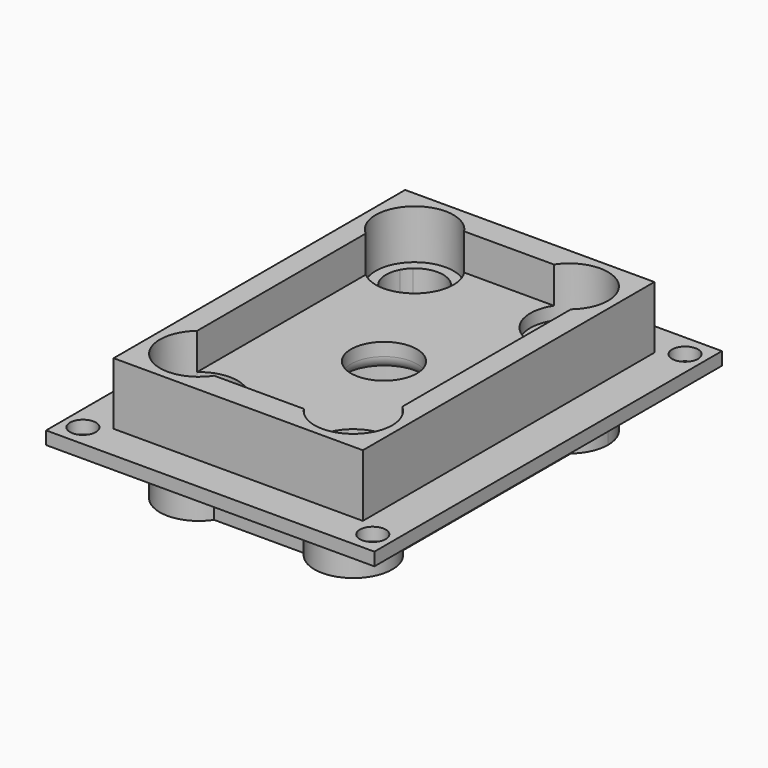
from build123d import *

# Parameters (mm, degrees)
F0_W      = 96.2
F0_H      = 140.65
F0_R      = 12.7
F1_DEPTH  = 5
F2_DEPTH  = 5
F3_DEPTH  = 19
F4_W      = 126.71781471
F4_H      = 167.6731868647
F4_R      = 5
F4_W_2    = 96.2
F4_H_2    = 140.65
F4_R_2    = 11
F4_R_3    = 30
F2_FACE_R = 12.7
F5_DEPTH  = 5
F6_DEPTH  = 30
F7_DEPTH  = 25
F8_R      = 12.7
F9_DEPTH  = 35
F4_R_4    = 12.7
F10_DEPTH = 35
F11_R     = 4.99999


# Not quite as in the source:
# - a fillet or chamfer is up to 0.001 mm smaller than in the source, because OpenCascade refuses the exact size


with BuildPart() as f1:
    # F0 (on Top) → F1 (new body)
    with BuildSketch(Plane.XY):
        with Locations((-2.6661262382, -2.1749504376)):
            Rectangle(F0_W, F0_H)
        with BuildLine():
            ThreePointArc((-42.2661262382, 38.498499743), (-42.4198102031, 61.1325113488), (-19.9826307497, 58.1500495624))
            Line((-19.9826307497, 58.1500495624), (14.6503782733, 58.1500495624))
            ThreePointArc((14.6503782733, 58.1500495624), (31.4825998108, 64.2478800491), (42.1661737618, 49.8823495624))
            ThreePointArc((42.1661737618, 49.8823495624), (40.7954712492, 43.6179860672), (36.9338737618, 38.498499743))
            Line((36.9338737618, 38.498499743), (36.9338737618, -42.8484006182))
            ThreePointArc((36.9338737618, -42.8484006182), (40.7954712492, -47.9678869424), (42.1661737618, -54.2322504376))
            ThreePointArc((42.1661737618, -54.2322504376), (31.4825998108, -68.5977809243), (14.6503782733, -62.4999504376))
            Line((14.6503782733, -62.4999504376), (-19.9826307497, -62.4999504376))
            ThreePointArc((-19.9826307497, -62.4999504376), (-42.4198102031, -65.482412224), (-42.2661262382, -42.8484006182))
            Line((-42.2661262382, -42.8484006182), (-42.2661262382, 38.498499743))
        make_face(mode=Mode.SUBTRACT)
        with BuildLine():
            Line((14.6503782733, 58.1500495624), (-19.9826307497, 58.1500495624))
            ThreePointArc((-19.9826307497, 58.1500495624), (-18.1328957515, 54.1987756114), (-17.4984262382, 49.8823495624))
            ThreePointArc((-17.4984262382, 49.8823495624), (-26.234062743, 36.253052075), (-42.2661262382, 38.498499743))
            Line((-42.2661262382, 38.498499743), (-42.2661262382, -42.8484006182))
            ThreePointArc((-42.2661262382, -42.8484006182), (-26.234062743, -40.6029529502), (-17.4984262382, -54.2322504376))
            ThreePointArc((-17.4984262382, -54.2322504376), (-18.1328957515, -58.5486764866), (-19.9826307497, -62.4999504376))
            Line((-19.9826307497, -62.4999504376), (14.6503782733, -62.4999504376))
            ThreePointArc((14.6503782733, -62.4999504376), (17.2447897969, -42.9820886512), (36.9338737618, -42.8484006182))
            Line((36.9338737618, -42.8484006182), (36.9338737618, 38.498499743))
            ThreePointArc((36.9338737618, 38.498499743), (17.2447897969, 38.632187776), (14.6503782733, 58.1500495624))
        make_face()
        with Locations((-2.6661262382, -2.1749504376)):
            Circle(F0_R, mode=Mode.SUBTRACT)
        with BuildLine():
            Line((-19.9826307497, 58.1500495624), (-25.2427293929, 58.1500495624))
            ThreePointArc((-25.2427293929, 58.1500495624), (-22.4781302022, 54.4203741713), (-21.4984262382, 49.8823495624))
            ThreePointArc((-21.4984262382, 49.8823495624), (-29.8950342201, 39.1948638899), (-42.2661262382, 44.823492309))
            Line((-42.2661262382, 44.823492309), (-42.2661262382, 38.498499743))
            ThreePointArc((-42.2661262382, 38.498499743), (-26.234062743, 36.253052075), (-17.4984262382, 49.8823495624))
            ThreePointArc((-17.4984262382, 49.8823495624), (-18.1328957515, 54.1987756114), (-19.9826307497, 58.1500495624))
        make_face()
        with BuildLine():
            Line((19.9104769166, 58.1500495624), (14.6503782733, 58.1500495624))
            ThreePointArc((14.6503782733, 58.1500495624), (17.2447897969, 38.632187776), (36.9338737618, 38.498499743))
            Line((36.9338737618, 38.498499743), (36.9338737618, 44.823492309))
            ThreePointArc((36.9338737618, 44.823492309), (20.3855526974, 41.2207574466), (19.9104769166, 58.1500495624))
        make_face()
        with BuildLine():
            ThreePointArc((-17.4984262382, -54.2322504376), (-26.234062743, -40.6029529502), (-42.2661262382, -42.8484006182))
            Line((-42.2661262382, -42.8484006182), (-42.2661262382, -49.1733931842))
            ThreePointArc((-42.2661262382, -49.1733931842), (-29.8950342201, -43.5447647651), (-21.4984262382, -54.2322504376))
            ThreePointArc((-21.4984262382, -54.2322504376), (-22.4781302022, -58.7702750465), (-25.2427293929, -62.4999504376))
            Line((-25.2427293929, -62.4999504376), (-19.9826307497, -62.4999504376))
            ThreePointArc((-19.9826307497, -62.4999504376), (-18.1328957515, -58.5486764866), (-17.4984262382, -54.2322504376))
        make_face()
        with BuildLine():
            Line((36.9338737618, -49.1733931842), (36.9338737618, -42.8484006182))
            ThreePointArc((36.9338737618, -42.8484006182), (17.2447897969, -42.9820886512), (14.6503782733, -62.4999504376))
            Line((14.6503782733, -62.4999504376), (19.9104769166, -62.4999504376))
            ThreePointArc((19.9104769166, -62.4999504376), (20.3855526974, -45.5706583218), (36.9338737618, -49.1733931842))
        make_face()
        with BuildLine():
            Line((-42.2661262382, 54.9412068158), (-42.2661262382, 58.1500495624))
            Line((-42.2661262382, 58.1500495624), (-39.7541230834, 58.1500495624))
            ThreePointArc((-39.7541230834, 58.1500495624), (-32.4984262382, 60.8823495624), (-25.2427293929, 58.1500495624))
            Line((-25.2427293929, 58.1500495624), (-19.9826307497, 58.1500495624))
            ThreePointArc((-19.9826307497, 58.1500495624), (-42.4198102031, 61.1325113488), (-42.2661262382, 38.498499743))
            Line((-42.2661262382, 38.498499743), (-42.2661262382, 44.823492309))
            ThreePointArc((-42.2661262382, 44.823492309), (-43.4984262382, 49.8823495624), (-42.2661262382, 54.9412068158))
        make_face()
        with BuildLine():
            ThreePointArc((42.1661737618, 49.8823495624), (31.4825998108, 64.2478800491), (14.6503782733, 58.1500495624))
            Line((14.6503782733, 58.1500495624), (19.9104769166, 58.1500495624))
            ThreePointArc((19.9104769166, 58.1500495624), (27.1661737618, 60.8823495624), (34.4218706071, 58.1500495624))
            Line((34.4218706071, 58.1500495624), (36.9338737618, 58.1500495624))
            Line((36.9338737618, 58.1500495624), (36.9338737618, 54.9412068158))
            ThreePointArc((36.9338737618, 54.9412068158), (37.8536594343, 52.4857415805), (38.1661737618, 49.8823495624))
            ThreePointArc((38.1661737618, 49.8823495624), (37.8536594343, 47.2789575443), (36.9338737618, 44.823492309))
            Line((36.9338737618, 44.823492309), (36.9338737618, 38.498499743))
            ThreePointArc((36.9338737618, 38.498499743), (40.7954712492, 43.6179860672), (42.1661737618, 49.8823495624))
        make_face()
        with BuildLine():
            Line((-42.2661262382, -49.1733931842), (-42.2661262382, -42.8484006182))
            ThreePointArc((-42.2661262382, -42.8484006182), (-42.4198102031, -65.482412224), (-19.9826307497, -62.4999504376))
            Line((-19.9826307497, -62.4999504376), (-25.2427293929, -62.4999504376))
            ThreePointArc((-25.2427293929, -62.4999504376), (-32.4984262382, -65.2322504376), (-39.7541230834, -62.4999504376))
            Line((-39.7541230834, -62.4999504376), (-42.2661262382, -62.4999504376))
            Line((-42.2661262382, -62.4999504376), (-42.2661262382, -59.291107691))
            ThreePointArc((-42.2661262382, -59.291107691), (-43.4984262382, -54.2322504376), (-42.2661262382, -49.1733931842))
        make_face()
        with BuildLine():
            ThreePointArc((42.1661737618, -54.2322504376), (40.7954712492, -47.9678869424), (36.9338737618, -42.8484006182))
            Line((36.9338737618, -42.8484006182), (36.9338737618, -49.1733931842))
            ThreePointArc((36.9338737618, -49.1733931842), (37.8536594343, -51.6288584195), (38.1661737618, -54.2322504376))
            ThreePointArc((38.1661737618, -54.2322504376), (37.8536594343, -56.8356424557), (36.9338737618, -59.291107691))
            Line((36.9338737618, -59.291107691), (36.9338737618, -62.4999504376))
            Line((36.9338737618, -62.4999504376), (34.4218706071, -62.4999504376))
            ThreePointArc((34.4218706071, -62.4999504376), (27.1661737618, -65.2322504376), (19.9104769166, -62.4999504376))
            Line((19.9104769166, -62.4999504376), (14.6503782733, -62.4999504376))
            ThreePointArc((14.6503782733, -62.4999504376), (31.4825998108, -68.5977809243), (42.1661737618, -54.2322504376))
        make_face()
        with BuildLine():
            Line((36.9338737618, 58.1500495624), (34.4218706071, 58.1500495624))
            ThreePointArc((34.4218706071, 58.1500495624), (35.8277658776, 56.6629706268), (36.9338737618, 54.9412068158))
            Line((36.9338737618, 54.9412068158), (36.9338737618, 58.1500495624))
        make_face()
        with BuildLine():
            Line((-39.7541230834, 58.1500495624), (-42.2661262382, 58.1500495624))
            Line((-42.2661262382, 58.1500495624), (-42.2661262382, 54.9412068158))
            ThreePointArc((-42.2661262382, 54.9412068158), (-41.160018354, 56.6629706268), (-39.7541230834, 58.1500495624))
        make_face()
        with BuildLine():
            Line((36.9338737618, -62.4999504376), (36.9338737618, -59.291107691))
            ThreePointArc((36.9338737618, -59.291107691), (35.8277658776, -61.012871502), (34.4218706071, -62.4999504376))
            Line((34.4218706071, -62.4999504376), (36.9338737618, -62.4999504376))
        make_face()
        with BuildLine():
            ThreePointArc((-39.7541230834, -62.4999504376), (-41.160018354, -61.012871502), (-42.2661262382, -59.291107691))
            Line((-42.2661262382, -59.291107691), (-42.2661262382, -62.4999504376))
            Line((-42.2661262382, -62.4999504376), (-39.7541230834, -62.4999504376))
        make_face()
    extrude(amount=-F1_DEPTH)

    # F0 (on Top) → F2 (join)
    with BuildSketch(Plane.XY):
        with BuildLine():
            Line((14.6503782733, 58.1500495624), (-19.9826307497, 58.1500495624))
            ThreePointArc((-19.9826307497, 58.1500495624), (-18.1328957515, 54.1987756114), (-17.4984262382, 49.8823495624))
            ThreePointArc((-17.4984262382, 49.8823495624), (-26.234062743, 36.253052075), (-42.2661262382, 38.498499743))
            Line((-42.2661262382, 38.498499743), (-42.2661262382, -42.8484006182))
            ThreePointArc((-42.2661262382, -42.8484006182), (-26.234062743, -40.6029529502), (-17.4984262382, -54.2322504376))
            ThreePointArc((-17.4984262382, -54.2322504376), (-18.1328957515, -58.5486764866), (-19.9826307497, -62.4999504376))
            Line((-19.9826307497, -62.4999504376), (14.6503782733, -62.4999504376))
            ThreePointArc((14.6503782733, -62.4999504376), (17.2447897969, -42.9820886512), (36.9338737618, -42.8484006182))
            Line((36.9338737618, -42.8484006182), (36.9338737618, 38.498499743))
            ThreePointArc((36.9338737618, 38.498499743), (17.2447897969, 38.632187776), (14.6503782733, 58.1500495624))
        make_face()
        with Locations((-2.6661262382, -2.1749504376)):
            Circle(F0_R, mode=Mode.SUBTRACT)
    extrude(amount=F2_DEPTH)

    # F0 (on Top) → F3 (join)
    with BuildSketch(Plane.XY):
        with Locations((-2.6661262382, -2.1749504376)):
            Rectangle(F0_W, F0_H)
        with BuildLine():
            ThreePointArc((-42.2661262382, 38.498499743), (-42.4198102031, 61.1325113488), (-19.9826307497, 58.1500495624))
            Line((-19.9826307497, 58.1500495624), (14.6503782733, 58.1500495624))
            ThreePointArc((14.6503782733, 58.1500495624), (31.4825998108, 64.2478800491), (42.1661737618, 49.8823495624))
            ThreePointArc((42.1661737618, 49.8823495624), (40.7954712492, 43.6179860672), (36.9338737618, 38.498499743))
            Line((36.9338737618, 38.498499743), (36.9338737618, -42.8484006182))
            ThreePointArc((36.9338737618, -42.8484006182), (40.7954712492, -47.9678869424), (42.1661737618, -54.2322504376))
            ThreePointArc((42.1661737618, -54.2322504376), (31.4825998108, -68.5977809243), (14.6503782733, -62.4999504376))
            Line((14.6503782733, -62.4999504376), (-19.9826307497, -62.4999504376))
            ThreePointArc((-19.9826307497, -62.4999504376), (-42.4198102031, -65.482412224), (-42.2661262382, -42.8484006182))
            Line((-42.2661262382, -42.8484006182), (-42.2661262382, 38.498499743))
        make_face(mode=Mode.SUBTRACT)
    extrude(amount=F3_DEPTH)

    # F4 (on face) + F2_face (on face) → F5 (join)
    with BuildSketch(Plane(origin=(0, 0, -5), x_dir=(1, 0, 0), z_dir=(0, 0, -1))):
        with Locations((-2.6661262382, 2.1749504376)):
            Rectangle(F4_W, F4_H)
        with Locations((-58.5996061093, -73.1500495624)):
            Circle(F4_R, mode=Mode.SUBTRACT)
        with Locations((53.2673536329, -73.1500495624)):
            Circle(F4_R, mode=Mode.SUBTRACT)
        with Locations((-2.6661262382, 2.1749504376)):
            Rectangle(F4_W_2, F4_H_2, mode=Mode.SUBTRACT)
        with Locations((-58.5996061093, 77.4999504376)):
            Circle(F4_R, mode=Mode.SUBTRACT)
        with Locations((53.2673536329, 77.4999504376)):
            Circle(F4_R, mode=Mode.SUBTRACT)
        with Locations((-2.6661262382, 2.1749504376)):
            Rectangle(F4_W_2, F4_H_2)
        with Locations((-32.4984262382, -49.8823495624)):
            Circle(F4_R_2, mode=Mode.SUBTRACT)
        with Locations((27.1661737618, -49.8823495624)):
            Circle(F4_R_2, mode=Mode.SUBTRACT)
        with Locations((-32.4984262382, 54.2322504376)):
            Circle(F4_R_2, mode=Mode.SUBTRACT)
        with Locations((-2.6661262382, 2.1749504376)):
            Circle(F4_R_3, mode=Mode.SUBTRACT)
        with Locations((27.1661737618, 54.2322504376)):
            Circle(F4_R_2, mode=Mode.SUBTRACT)
    with BuildSketch(Plane(origin=(-2.6661262382, -2.1749504376, 5), x_dir=(1, 0, 0), z_dir=(0, 0, 1))):
        with BuildLine():
            Line((17.3165045115, 60.325), (-17.3165045115, 60.325))
            ThreePointArc((-17.3165045115, 60.325), (-19.9109160351, 40.8071382136), (-39.6, 40.6734501806))
            Line((-39.6, 40.6734501806), (-39.6, -40.6734501806))
            ThreePointArc((-39.6, -40.6734501806), (-19.9109160351, -40.8071382136), (-17.3165045115, -60.325))
            Line((-17.3165045115, -60.325), (17.3165045115, -60.325))
            ThreePointArc((17.3165045115, -60.325), (19.9109160351, -40.8071382136), (39.6, -40.6734501806))
            Line((39.6, -40.6734501806), (39.6, 40.6734501806))
            ThreePointArc((39.6, 40.6734501806), (19.9109160351, 40.8071382136), (17.3165045115, 60.325))
        make_face()
        Circle(F2_FACE_R, mode=Mode.SUBTRACT)
    extrude(amount=F5_DEPTH, dir=(0, 0, -1))

    # F0 (on Top) → F6 (join)
    with BuildSketch(Plane.XY):
        with BuildLine():
            Line((-42.2661262382, 54.9412068158), (-42.2661262382, 58.1500495624))
            Line((-42.2661262382, 58.1500495624), (-39.7541230834, 58.1500495624))
            ThreePointArc((-39.7541230834, 58.1500495624), (-32.4984262382, 60.8823495624), (-25.2427293929, 58.1500495624))
            Line((-25.2427293929, 58.1500495624), (-19.9826307497, 58.1500495624))
            ThreePointArc((-19.9826307497, 58.1500495624), (-42.4198102031, 61.1325113488), (-42.2661262382, 38.498499743))
            Line((-42.2661262382, 38.498499743), (-42.2661262382, 44.823492309))
            ThreePointArc((-42.2661262382, 44.823492309), (-43.4984262382, 49.8823495624), (-42.2661262382, 54.9412068158))
        make_face()
        with BuildLine():
            ThreePointArc((-25.2427293929, 58.1500495624), (-32.4984262382, 60.8823495624), (-39.7541230834, 58.1500495624))
            Line((-39.7541230834, 58.1500495624), (-25.2427293929, 58.1500495624))
        make_face()
        with BuildLine():
            Line((-39.7541230834, 58.1500495624), (-42.2661262382, 58.1500495624))
            Line((-42.2661262382, 58.1500495624), (-42.2661262382, 54.9412068158))
            ThreePointArc((-42.2661262382, 54.9412068158), (-41.160018354, 56.6629706268), (-39.7541230834, 58.1500495624))
        make_face()
        with BuildLine():
            Line((-42.2661262382, 44.823492309), (-42.2661262382, 54.9412068158))
            ThreePointArc((-42.2661262382, 54.9412068158), (-43.4984262382, 49.8823495624), (-42.2661262382, 44.823492309))
        make_face()
        with BuildLine():
            Line((-19.9826307497, 58.1500495624), (-25.2427293929, 58.1500495624))
            ThreePointArc((-25.2427293929, 58.1500495624), (-22.4781302022, 54.4203741713), (-21.4984262382, 49.8823495624))
            ThreePointArc((-21.4984262382, 49.8823495624), (-29.8950342201, 39.1948638899), (-42.2661262382, 44.823492309))
            Line((-42.2661262382, 44.823492309), (-42.2661262382, 38.498499743))
            ThreePointArc((-42.2661262382, 38.498499743), (-26.234062743, 36.253052075), (-17.4984262382, 49.8823495624))
            ThreePointArc((-17.4984262382, 49.8823495624), (-18.1328957515, 54.1987756114), (-19.9826307497, 58.1500495624))
        make_face()
        with BuildLine():
            Line((-25.2427293929, 58.1500495624), (-39.7541230834, 58.1500495624))
            ThreePointArc((-39.7541230834, 58.1500495624), (-41.160018354, 56.6629706268), (-42.2661262382, 54.9412068158))
            Line((-42.2661262382, 54.9412068158), (-42.2661262382, 44.823492309))
            ThreePointArc((-42.2661262382, 44.823492309), (-29.8950342201, 39.1948638899), (-21.4984262382, 49.8823495624))
            ThreePointArc((-21.4984262382, 49.8823495624), (-22.4781302022, 54.4203741713), (-25.2427293929, 58.1500495624))
        make_face()
        with BuildLine():
            ThreePointArc((42.1661737618, 49.8823495624), (31.4825998108, 64.2478800491), (14.6503782733, 58.1500495624))
            Line((14.6503782733, 58.1500495624), (19.9104769166, 58.1500495624))
            ThreePointArc((19.9104769166, 58.1500495624), (27.1661737618, 60.8823495624), (34.4218706071, 58.1500495624))
            Line((34.4218706071, 58.1500495624), (36.9338737618, 58.1500495624))
            Line((36.9338737618, 58.1500495624), (36.9338737618, 54.9412068158))
            ThreePointArc((36.9338737618, 54.9412068158), (37.8536594343, 52.4857415805), (38.1661737618, 49.8823495624))
            ThreePointArc((38.1661737618, 49.8823495624), (37.8536594343, 47.2789575443), (36.9338737618, 44.823492309))
            Line((36.9338737618, 44.823492309), (36.9338737618, 38.498499743))
            ThreePointArc((36.9338737618, 38.498499743), (40.7954712492, 43.6179860672), (42.1661737618, 49.8823495624))
        make_face()
        with BuildLine():
            Line((36.9338737618, 54.9412068158), (36.9338737618, 44.823492309))
            ThreePointArc((36.9338737618, 44.823492309), (37.8536594343, 47.2789575443), (38.1661737618, 49.8823495624))
            ThreePointArc((38.1661737618, 49.8823495624), (37.8536594343, 52.4857415805), (36.9338737618, 54.9412068158))
        make_face()
        with BuildLine():
            Line((34.4218706071, 58.1500495624), (19.9104769166, 58.1500495624))
            ThreePointArc((19.9104769166, 58.1500495624), (20.3855526974, 41.2207574466), (36.9338737618, 44.823492309))
            Line((36.9338737618, 44.823492309), (36.9338737618, 54.9412068158))
            ThreePointArc((36.9338737618, 54.9412068158), (35.8277658776, 56.6629706268), (34.4218706071, 58.1500495624))
        make_face()
        with BuildLine():
            Line((36.9338737618, 58.1500495624), (34.4218706071, 58.1500495624))
            ThreePointArc((34.4218706071, 58.1500495624), (35.8277658776, 56.6629706268), (36.9338737618, 54.9412068158))
            Line((36.9338737618, 54.9412068158), (36.9338737618, 58.1500495624))
        make_face()
        with BuildLine():
            ThreePointArc((34.4218706071, 58.1500495624), (27.1661737618, 60.8823495624), (19.9104769166, 58.1500495624))
            Line((19.9104769166, 58.1500495624), (34.4218706071, 58.1500495624))
        make_face()
        with BuildLine():
            Line((19.9104769166, 58.1500495624), (14.6503782733, 58.1500495624))
            ThreePointArc((14.6503782733, 58.1500495624), (17.2447897969, 38.632187776), (36.9338737618, 38.498499743))
            Line((36.9338737618, 38.498499743), (36.9338737618, 44.823492309))
            ThreePointArc((36.9338737618, 44.823492309), (20.3855526974, 41.2207574466), (19.9104769166, 58.1500495624))
        make_face()
        with BuildLine():
            ThreePointArc((42.1661737618, -54.2322504376), (40.7954712492, -47.9678869424), (36.9338737618, -42.8484006182))
            Line((36.9338737618, -42.8484006182), (36.9338737618, -49.1733931842))
            ThreePointArc((36.9338737618, -49.1733931842), (37.8536594343, -51.6288584195), (38.1661737618, -54.2322504376))
            ThreePointArc((38.1661737618, -54.2322504376), (37.8536594343, -56.8356424557), (36.9338737618, -59.291107691))
            Line((36.9338737618, -59.291107691), (36.9338737618, -62.4999504376))
            Line((36.9338737618, -62.4999504376), (34.4218706071, -62.4999504376))
            ThreePointArc((34.4218706071, -62.4999504376), (27.1661737618, -65.2322504376), (19.9104769166, -62.4999504376))
            Line((19.9104769166, -62.4999504376), (14.6503782733, -62.4999504376))
            ThreePointArc((14.6503782733, -62.4999504376), (31.4825998108, -68.5977809243), (42.1661737618, -54.2322504376))
        make_face()
        with BuildLine():
            Line((36.9338737618, -49.1733931842), (36.9338737618, -42.8484006182))
            ThreePointArc((36.9338737618, -42.8484006182), (17.2447897969, -42.9820886512), (14.6503782733, -62.4999504376))
            Line((14.6503782733, -62.4999504376), (19.9104769166, -62.4999504376))
            ThreePointArc((19.9104769166, -62.4999504376), (20.3855526974, -45.5706583218), (36.9338737618, -49.1733931842))
        make_face()
        with BuildLine():
            Line((36.9338737618, -59.291107691), (36.9338737618, -49.1733931842))
            ThreePointArc((36.9338737618, -49.1733931842), (20.3855526974, -45.5706583218), (19.9104769166, -62.4999504376))
            Line((19.9104769166, -62.4999504376), (34.4218706071, -62.4999504376))
            ThreePointArc((34.4218706071, -62.4999504376), (35.8277658776, -61.012871502), (36.9338737618, -59.291107691))
        make_face()
        with BuildLine():
            Line((34.4218706071, -62.4999504376), (19.9104769166, -62.4999504376))
            ThreePointArc((19.9104769166, -62.4999504376), (27.1661737618, -65.2322504376), (34.4218706071, -62.4999504376))
        make_face()
        with BuildLine():
            ThreePointArc((38.1661737618, -54.2322504376), (37.8536594343, -51.6288584195), (36.9338737618, -49.1733931842))
            Line((36.9338737618, -49.1733931842), (36.9338737618, -59.291107691))
            ThreePointArc((36.9338737618, -59.291107691), (37.8536594343, -56.8356424557), (38.1661737618, -54.2322504376))
        make_face()
        with BuildLine():
            Line((36.9338737618, -62.4999504376), (36.9338737618, -59.291107691))
            ThreePointArc((36.9338737618, -59.291107691), (35.8277658776, -61.012871502), (34.4218706071, -62.4999504376))
            Line((34.4218706071, -62.4999504376), (36.9338737618, -62.4999504376))
        make_face()
        with BuildLine():
            Line((-42.2661262382, -49.1733931842), (-42.2661262382, -42.8484006182))
            ThreePointArc((-42.2661262382, -42.8484006182), (-42.4198102031, -65.482412224), (-19.9826307497, -62.4999504376))
            Line((-19.9826307497, -62.4999504376), (-25.2427293929, -62.4999504376))
            ThreePointArc((-25.2427293929, -62.4999504376), (-32.4984262382, -65.2322504376), (-39.7541230834, -62.4999504376))
            Line((-39.7541230834, -62.4999504376), (-42.2661262382, -62.4999504376))
            Line((-42.2661262382, -62.4999504376), (-42.2661262382, -59.291107691))
            ThreePointArc((-42.2661262382, -59.291107691), (-43.4984262382, -54.2322504376), (-42.2661262382, -49.1733931842))
        make_face()
        with BuildLine():
            ThreePointArc((-17.4984262382, -54.2322504376), (-26.234062743, -40.6029529502), (-42.2661262382, -42.8484006182))
            Line((-42.2661262382, -42.8484006182), (-42.2661262382, -49.1733931842))
            ThreePointArc((-42.2661262382, -49.1733931842), (-29.8950342201, -43.5447647651), (-21.4984262382, -54.2322504376))
            ThreePointArc((-21.4984262382, -54.2322504376), (-22.4781302022, -58.7702750465), (-25.2427293929, -62.4999504376))
            Line((-25.2427293929, -62.4999504376), (-19.9826307497, -62.4999504376))
            ThreePointArc((-19.9826307497, -62.4999504376), (-18.1328957515, -58.5486764866), (-17.4984262382, -54.2322504376))
        make_face()
        with BuildLine():
            ThreePointArc((-21.4984262382, -54.2322504376), (-29.8950342201, -43.5447647651), (-42.2661262382, -49.1733931842))
            Line((-42.2661262382, -49.1733931842), (-42.2661262382, -59.291107691))
            ThreePointArc((-42.2661262382, -59.291107691), (-41.160018354, -61.012871502), (-39.7541230834, -62.4999504376))
            Line((-39.7541230834, -62.4999504376), (-25.2427293929, -62.4999504376))
            ThreePointArc((-25.2427293929, -62.4999504376), (-22.4781302022, -58.7702750465), (-21.4984262382, -54.2322504376))
        make_face()
        with BuildLine():
            Line((-42.2661262382, -59.291107691), (-42.2661262382, -49.1733931842))
            ThreePointArc((-42.2661262382, -49.1733931842), (-43.4984262382, -54.2322504376), (-42.2661262382, -59.291107691))
        make_face()
        with BuildLine():
            ThreePointArc((-39.7541230834, -62.4999504376), (-41.160018354, -61.012871502), (-42.2661262382, -59.291107691))
            Line((-42.2661262382, -59.291107691), (-42.2661262382, -62.4999504376))
            Line((-42.2661262382, -62.4999504376), (-39.7541230834, -62.4999504376))
        make_face()
        with BuildLine():
            ThreePointArc((-39.7541230834, -62.4999504376), (-32.4984262382, -65.2322504376), (-25.2427293929, -62.4999504376))
            Line((-25.2427293929, -62.4999504376), (-39.7541230834, -62.4999504376))
        make_face()
        with BuildLine():
            Line((14.6503782733, 58.1500495624), (-19.9826307497, 58.1500495624))
            ThreePointArc((-19.9826307497, 58.1500495624), (-18.1328957515, 54.1987756114), (-17.4984262382, 49.8823495624))
            ThreePointArc((-17.4984262382, 49.8823495624), (-26.234062743, 36.253052075), (-42.2661262382, 38.498499743))
            Line((-42.2661262382, 38.498499743), (-42.2661262382, -42.8484006182))
            ThreePointArc((-42.2661262382, -42.8484006182), (-26.234062743, -40.6029529502), (-17.4984262382, -54.2322504376))
            ThreePointArc((-17.4984262382, -54.2322504376), (-18.1328957515, -58.5486764866), (-19.9826307497, -62.4999504376))
            Line((-19.9826307497, -62.4999504376), (14.6503782733, -62.4999504376))
            ThreePointArc((14.6503782733, -62.4999504376), (17.2447897969, -42.9820886512), (36.9338737618, -42.8484006182))
            Line((36.9338737618, -42.8484006182), (36.9338737618, 38.498499743))
            ThreePointArc((36.9338737618, 38.498499743), (17.2447897969, 38.632187776), (14.6503782733, 58.1500495624))
        make_face()
        with Locations((-2.6661262382, -2.1749504376)):
            Circle(F0_R, mode=Mode.SUBTRACT)
        with Locations((-2.6661262382, -2.1749504376)):
            Circle(F0_R)
    extrude(amount=-F6_DEPTH)

    # F0 (on Top) → F7 (cut)
    with BuildSketch(Plane.XY):
        with BuildLine():
            Line((34.4218706071, 58.1500495624), (19.9104769166, 58.1500495624))
            ThreePointArc((19.9104769166, 58.1500495624), (20.3855526974, 41.2207574466), (36.9338737618, 44.823492309))
            Line((36.9338737618, 44.823492309), (36.9338737618, 54.9412068158))
            ThreePointArc((36.9338737618, 54.9412068158), (35.8277658776, 56.6629706268), (34.4218706071, 58.1500495624))
        make_face()
        with BuildLine():
            ThreePointArc((34.4218706071, 58.1500495624), (27.1661737618, 60.8823495624), (19.9104769166, 58.1500495624))
            Line((19.9104769166, 58.1500495624), (34.4218706071, 58.1500495624))
        make_face()
        with BuildLine():
            Line((36.9338737618, 54.9412068158), (36.9338737618, 44.823492309))
            ThreePointArc((36.9338737618, 44.823492309), (37.8536594343, 47.2789575443), (38.1661737618, 49.8823495624))
            ThreePointArc((38.1661737618, 49.8823495624), (37.8536594343, 52.4857415805), (36.9338737618, 54.9412068158))
        make_face()
        with BuildLine():
            Line((-25.2427293929, 58.1500495624), (-39.7541230834, 58.1500495624))
            ThreePointArc((-39.7541230834, 58.1500495624), (-41.160018354, 56.6629706268), (-42.2661262382, 54.9412068158))
            Line((-42.2661262382, 54.9412068158), (-42.2661262382, 44.823492309))
            ThreePointArc((-42.2661262382, 44.823492309), (-29.8950342201, 39.1948638899), (-21.4984262382, 49.8823495624))
            ThreePointArc((-21.4984262382, 49.8823495624), (-22.4781302022, 54.4203741713), (-25.2427293929, 58.1500495624))
        make_face()
        with BuildLine():
            ThreePointArc((-25.2427293929, 58.1500495624), (-32.4984262382, 60.8823495624), (-39.7541230834, 58.1500495624))
            Line((-39.7541230834, 58.1500495624), (-25.2427293929, 58.1500495624))
        make_face()
        with BuildLine():
            Line((-42.2661262382, 44.823492309), (-42.2661262382, 54.9412068158))
            ThreePointArc((-42.2661262382, 54.9412068158), (-43.4984262382, 49.8823495624), (-42.2661262382, 44.823492309))
        make_face()
        with BuildLine():
            Line((36.9338737618, -59.291107691), (36.9338737618, -49.1733931842))
            ThreePointArc((36.9338737618, -49.1733931842), (20.3855526974, -45.5706583218), (19.9104769166, -62.4999504376))
            Line((19.9104769166, -62.4999504376), (34.4218706071, -62.4999504376))
            ThreePointArc((34.4218706071, -62.4999504376), (35.8277658776, -61.012871502), (36.9338737618, -59.291107691))
        make_face()
        with BuildLine():
            ThreePointArc((38.1661737618, -54.2322504376), (37.8536594343, -51.6288584195), (36.9338737618, -49.1733931842))
            Line((36.9338737618, -49.1733931842), (36.9338737618, -59.291107691))
            ThreePointArc((36.9338737618, -59.291107691), (37.8536594343, -56.8356424557), (38.1661737618, -54.2322504376))
        make_face()
        with BuildLine():
            Line((34.4218706071, -62.4999504376), (19.9104769166, -62.4999504376))
            ThreePointArc((19.9104769166, -62.4999504376), (27.1661737618, -65.2322504376), (34.4218706071, -62.4999504376))
        make_face()
        with BuildLine():
            ThreePointArc((-21.4984262382, -54.2322504376), (-29.8950342201, -43.5447647651), (-42.2661262382, -49.1733931842))
            Line((-42.2661262382, -49.1733931842), (-42.2661262382, -59.291107691))
            ThreePointArc((-42.2661262382, -59.291107691), (-41.160018354, -61.012871502), (-39.7541230834, -62.4999504376))
            Line((-39.7541230834, -62.4999504376), (-25.2427293929, -62.4999504376))
            ThreePointArc((-25.2427293929, -62.4999504376), (-22.4781302022, -58.7702750465), (-21.4984262382, -54.2322504376))
        make_face()
        with BuildLine():
            Line((-42.2661262382, -59.291107691), (-42.2661262382, -49.1733931842))
            ThreePointArc((-42.2661262382, -49.1733931842), (-43.4984262382, -54.2322504376), (-42.2661262382, -59.291107691))
        make_face()
        with BuildLine():
            ThreePointArc((-39.7541230834, -62.4999504376), (-32.4984262382, -65.2322504376), (-25.2427293929, -62.4999504376))
            Line((-25.2427293929, -62.4999504376), (-39.7541230834, -62.4999504376))
        make_face()
    extrude(amount=-F7_DEPTH, mode=Mode.SUBTRACT)

    # F8 (on face) → F9 (cut)
    with BuildSketch(Plane.XY):
        with Locations((-2.6661262382, -2.1749504376)):
            Circle(F8_R)
    extrude(amount=-F9_DEPTH, mode=Mode.SUBTRACT)

    # F4 (on face) → F10 (cut)
    with BuildSketch(Plane(origin=(0, 0, -5), x_dir=(1, 0, 0), z_dir=(0, 0, -1))):
        with Locations((-2.6661262382, 2.1749504376)):
            Circle(F4_R_3)
        with Locations((-2.6661262382, 2.1749504376)):
            Circle(F4_R_4, mode=Mode.SUBTRACT)
    extrude(amount=F10_DEPTH, mode=Mode.SUBTRACT)

    # F11 (radius 5 in the source; OpenCascade refuses exactly that, so slightly less here)
    f11_edges = [f1.edges().sort_by_distance(p)[0] for p in [
        (-32.666126, -2.17495, -5),
        (-15.366126, -2.17495, -5),
    ]]
    fillet(f11_edges, radius=F11_R)


solid = f1.part
